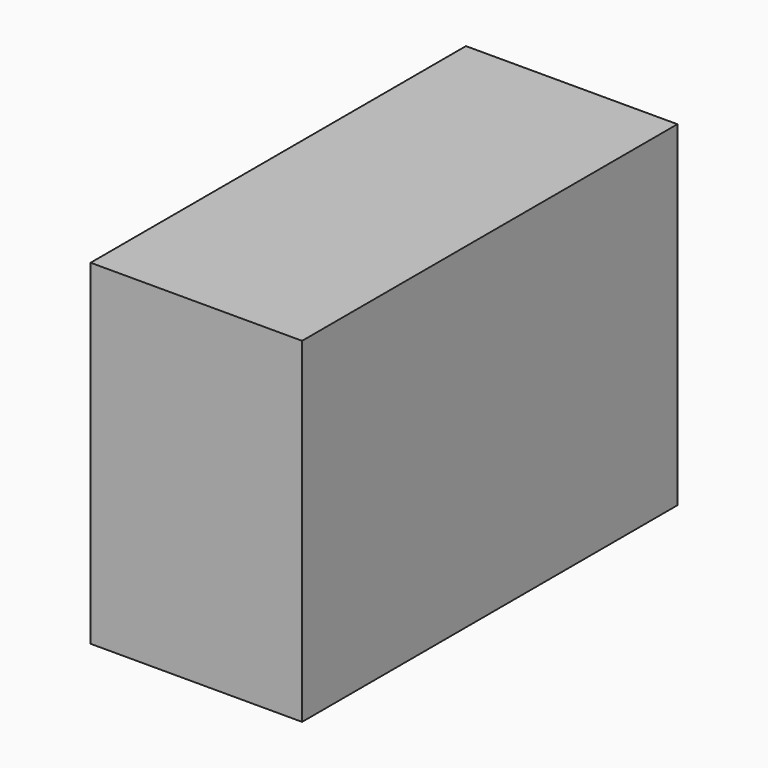
from build123d import *

# Parameters (mm, degrees)
F1_DEPTH = 2


# Not quite as in the source:
# - a feature names something its author has since deleted; it is built from what else it names


with BuildPart() as f1:
    # F0 (on Front) → F1 (new body)
    with BuildSketch(Plane.XZ):
        Polygon((-19.5010053796, 7.7693229541), (-19.5010053796, 8.4021232677), (-19.5010053796, 9.1995391995), (-20.4025600106, 9.1995391995), (-20.4025600106, 7.7693229541), align=None)
    extrude(amount=F1_DEPTH)


solid = f1.part
